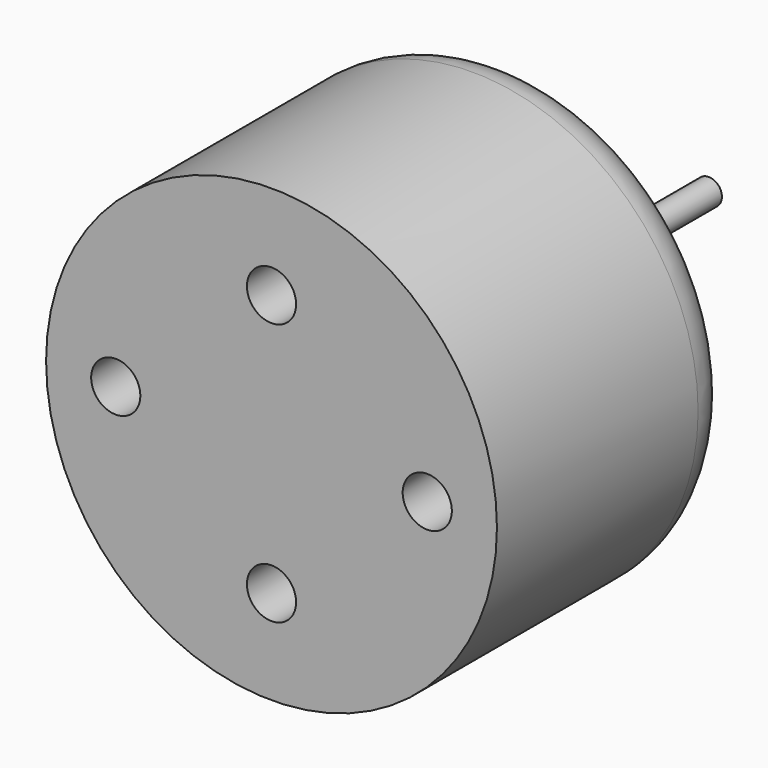
from build123d import *

# Parameters (mm, degrees)
F0_R     = 13.75
F0_R_2   = 1.5
F1_DEPTH = 18.34
F2_R     = 5
F3_DEPTH = 1
F4_R     = 0.8
F5_DEPTH = 15


# Not quite as in the source:
# - a fillet or chamfer that OpenCascade refuses, or shapes differently, is made with other operations: its cross-section is extruded or revolved along the edge and cut away or added


with BuildPart() as f1:
    # F0 (on Front) → F1 (new body)
    with BuildSketch(Plane.XZ):
        Circle(F0_R)
        with Locations((0, -8)):
            Circle(F0_R_2, mode=Mode.SUBTRACT)
        with Locations((-9.5, 0)):
            Circle(F0_R_2, mode=Mode.SUBTRACT)
        with Locations((9.5, 0)):
            Circle(F0_R_2, mode=Mode.SUBTRACT)
        with Locations((0, 8)):
            Circle(F0_R_2, mode=Mode.SUBTRACT)
    extrude(amount=F1_DEPTH)

    # F2 (on Front) → F3 (join)
    with BuildSketch(Plane.XZ):
        Circle(F2_R)
    extrude(amount=-F3_DEPTH)

    # F4 (on Front) → F5 (join)
    with BuildSketch(Plane.XZ):
        Circle(F4_R)
    extrude(amount=-F5_DEPTH)

    # F6: fillet of radius 3 on 1 edges, made by hand

    # F6_s1 → F6_t2 (revolve, cut)
    with BuildSketch(Plane.XY):
        with BuildLine():
            ThreePointArc((13.75, -3), (12.8713203436, -0.8786796564), (10.75, 0))
            Line((10.75, 0), (13.75, 0))
            Line((13.75, 0), (13.75, -3))
        make_face()
    revolve(axis=Axis((0, 0, 0), (0, -1, 0)), mode=Mode.SUBTRACT)


solid = f1.part
